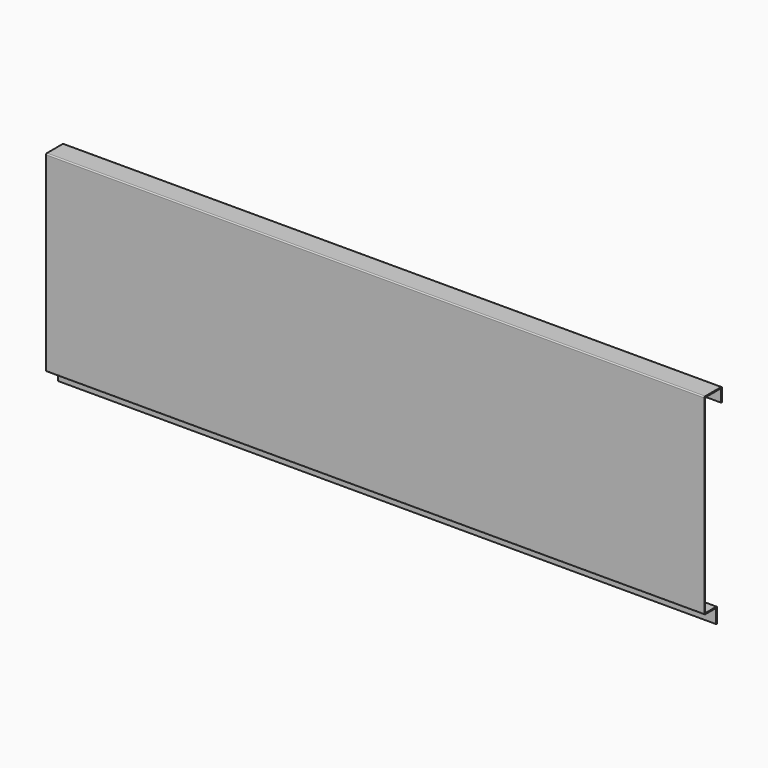
from build123d import *

# Parameters (mm, degrees)
F1_DEPTH = 1200
F3_D     = 5
F4_R     = 2


# Not quite as in the source:
# - a feature names something its author has since deleted; it is built from what else it names


with BuildPart() as f1:
    # F0 (on Right) → F1 (new body)
    with BuildSketch(Plane.YZ):
        Polygon((-18.8378913403, 427.8021101952), (-18.8378913403, 404.8021101952), (-16.8378913403, 404.8021101952), (-16.8378913403, 429.8021101952), (-56.8378913403, 429.8021101952), (-56.8378913403, 79.8021101952), (-29.8378913403, 79.8021101952), (-29.8378913403, 53.8021101952), (-27.8378913403, 53.8021101952), (-27.8378913403, 81.8021101952), (-54.8378913403, 81.8021101952), (-54.8378913403, 427.8021101952), align=None)
    extrude(amount=F1_DEPTH)

    # F3 (through all)
    with Locations(Plane.XZ.offset(29.8378913403)):
        with Locations((433, 66.8021101952), (767, 66.8021101952), (1100, 66.8021101952), (100, 66.8021101952)):
            Hole(F3_D / 2)

    # F4
    f4_edges = [f1.edges().sort_by_distance(p)[0] for p in [
        (600, -56.837891, 429.80211),
        (600, -16.837891, 429.80211),
        (600, -56.837891, 79.80211),
        (600, -27.837891, 81.80211),
        (600, -54.837891, 81.80211),
        (600, -29.837891, 79.80211),
        (600, -18.837891, 427.80211),
        (600, -54.837891, 427.80211),
    ]]
    fillet(f4_edges, radius=F4_R)


solid = f1.part
